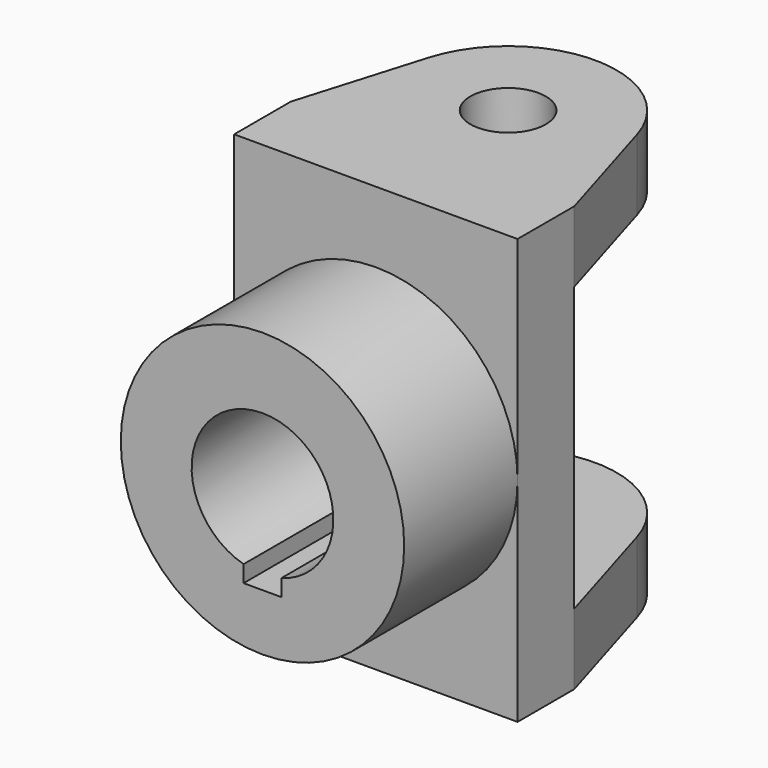
from build123d import *

# Parameters (mm, degrees)
F0_W     = 60
F0_H     = 90
F1_DEPTH = 15
F2_R     = 30
F3_DEPTH = 30
F4_R     = 8
F5_DEPTH = 15


# Not quite as in the source:
# - a pattern or mirror of a feature is missing from the dataset's text; its kind, count and spacing are read off the source's solid


with BuildPart() as f1:
    # F0 (on Front) → F1 (new body)
    with BuildSketch(Plane.XZ):
        Rectangle(F0_W, F0_H)
    extrude(amount=F1_DEPTH)

    # F2 (on face) → F3 (join)
    with BuildSketch(Plane.XZ.offset(15)):
        Circle(F2_R)
        with BuildLine():
            ThreePointArc((-4, -14.4568322948), (0, 15), (4, -14.4568322948))
            Line((4, -14.4568322948), (4, -18))
            Line((4, -18), (0, -18))
            Line((0, -18), (-4, -18))
            Line((-4, -18), (-4, -14.4568322948))
        make_face(mode=Mode.SUBTRACT)
    extrude(amount=F3_DEPTH)

    # F4 (on face) → F5 (join)
    with BuildSketch(Plane.XY.offset(45)):
        with BuildLine():
            Line((30, 0), (22.0328983898, 26.5993475847))
            ThreePointArc((22.0328983898, 26.5993475847), (0, 43), (-22.0328983898, 26.5993475847))
            Line((-22.0328983898, 26.5993475847), (-30, 0))
            Line((-30, 0), (30, 0))
        make_face()
        with Locations((0, 20)):
            Circle(F4_R, mode=Mode.SUBTRACT)
    f5 = extrude(amount=-F5_DEPTH)

    # F5_copies: F5 across plane
    add(f5.mirror(Plane(origin=(0, 0, 0), x_dir=(-1, 0, 0), z_dir=(0, 0, -1))))


solid = f1.part
